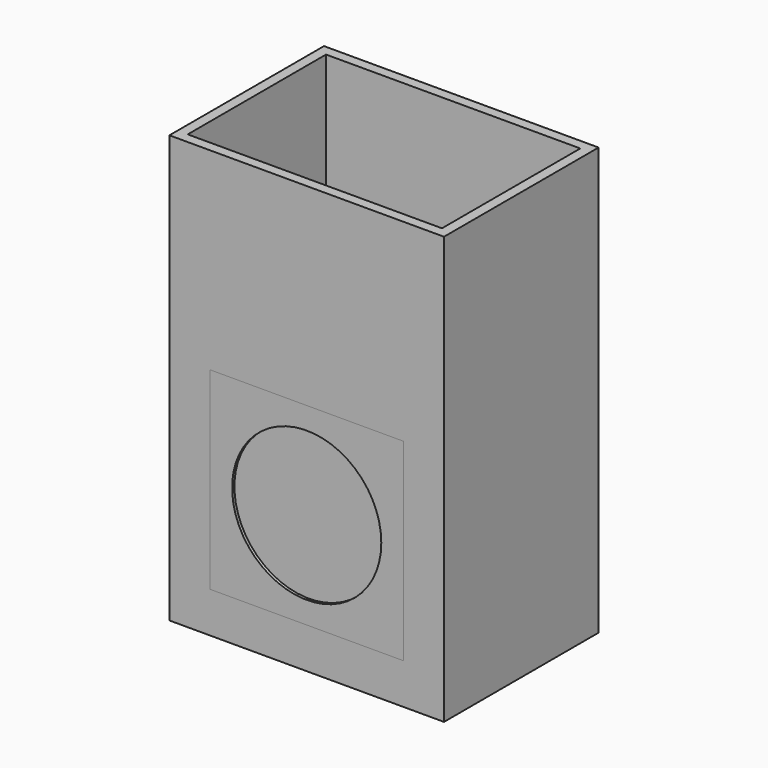
from build123d import *

# Parameters (mm, degrees)
F0_W      = 120.65
F0_H      = 120.65
F1_DEPTH  = 120.65
F2_R      = 46.5747584451
F3_DEPTH  = 1.778
F5_W      = 171.45
F5_H      = 120.65
F6_DEPTH  = 25.4
F7_W      = 25.4
F7_H      = 120.65
F8_DEPTH  = 120.65
F9_DEPTH  = 120.65
F10_W     = 120.65
F10_H     = 120.65
F11_DEPTH = 120.65
F12_T     = -6.35


with BuildPart() as f1:
    # F0 (on Top) → F1 (new body)
    with BuildSketch(Plane.XY):
        Rectangle(F0_W, F0_H)
    extrude(amount=F1_DEPTH)

    # F2 (on face) → F3 (cut)
    with BuildSketch(Plane.XZ.offset(60.325)):
        with Locations((0, 60.325)):
            Circle(F2_R)
    extrude(amount=-F3_DEPTH, mode=Mode.SUBTRACT)


with BuildPart() as f1_1:
    # F4: moved
    add(f1.part.moved(Location((0, 0, 25.4))))


with BuildPart() as f6:
    # F5 (on Top) → F6 (new body)
    with BuildSketch(Plane.XY):
        Rectangle(F5_W, F5_H)
    extrude(amount=F6_DEPTH)

    # F7 (on face) → F8 (join)
    with BuildSketch(Plane.XY.offset(25.4)):
        with Locations((-73.025, 0)):
            Rectangle(F7_W, F7_H)
        with Locations((73.025, 0)):
            Rectangle(F7_W, F7_H)
    extrude(amount=F8_DEPTH)

    # F9 (add): faces of the model
    f9_faces = [f6.faces().sort_by_distance(p)[0] for p in [
        (-73.025, 0, 146.05),
        (73.025, 0, 146.05),
    ]]
    extrude(f9_faces, amount=F9_DEPTH)

    # F10 (on face) → F11 (join)
    with BuildSketch(Plane.YZ.offset(-60.325)):
        with Locations((0, 206.375)):
            Rectangle(F10_W, F10_H)
    extrude(amount=F11_DEPTH)

    # F12
    f12_openings = [f6.faces().sort_by_distance(p)[0] for p in [
        (0, 0, 266.7),
    ]]
    offset(amount=F12_T, openings=f12_openings, kind=Kind.INTERSECTION)


solid = Compound([f1_1.part, f6.part])
